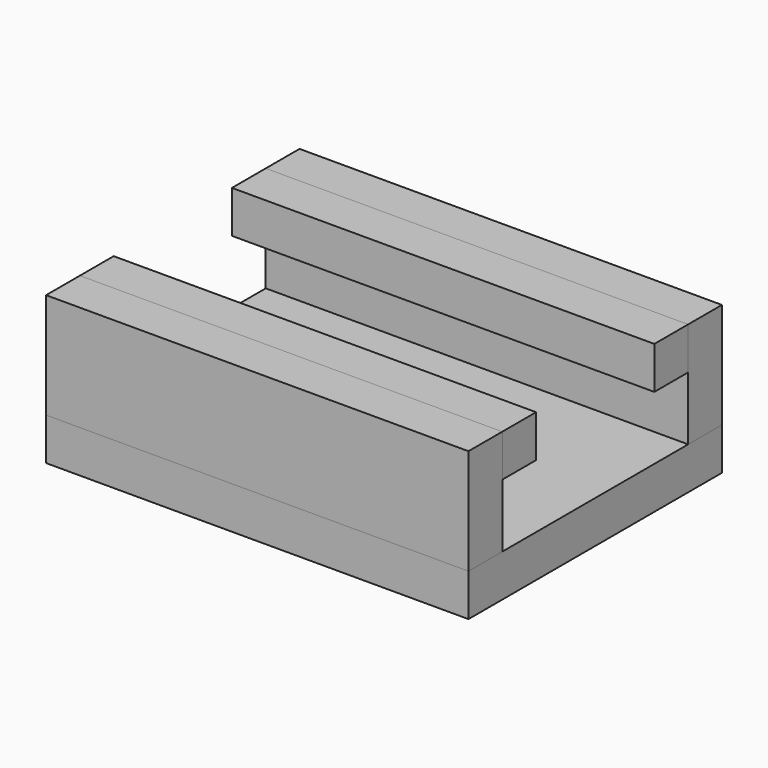
from build123d import *

# Parameters (mm, degrees)
F0_W     = 20
F0_H     = 2
F1_DEPTH = 7
F0_H_2   = 7
F2_DEPTH = 2
F3_START = 5
F3_DEPTH = 2


with BuildPart() as f1:
    # F0 (on Top) → F1 (new body)
    with BuildSketch(Plane.XY):
        with Locations((-33.0076411562, -6.5)):
            Rectangle(F0_W, F0_H)
    extrude(amount=F1_DEPTH)


with BuildPart() as f1b:
    # F0 (on Top) → F1, piece 2 (new body)
    with BuildSketch(Plane.XY):
        with Locations((-33.0076411562, 6.5)):
            Rectangle(F0_W, F0_H)
    extrude(amount=F1_DEPTH)


with BuildPart() as f2:
    # F0 (on Top) → F2 (new body)
    with BuildSketch(Plane.XY):
        with Locations((-33.0076411562, 6.5)):
            Rectangle(F0_W, F0_H)
        with Locations((-33.0076411562, 4.5)):
            Rectangle(F0_W, F0_H)
        with Locations((-33.0076411562, 0)):
            Rectangle(F0_W, F0_H_2)
        with Locations((-33.0076411562, -4.5)):
            Rectangle(F0_W, F0_H)
        with Locations((-33.0076411562, -6.5)):
            Rectangle(F0_W, F0_H)
    extrude(amount=F2_DEPTH)


with BuildPart() as f3:
    # F0 (on Top) → F3 (new body)
    with BuildSketch(Plane.XY.offset(F3_START)):
        with Locations((-33.0076411562, 4.5)):
            Rectangle(F0_W, F0_H)
    extrude(amount=F3_DEPTH)


with BuildPart() as f3b:
    # F0 (on Top) → F3, piece 2 (new body)
    with BuildSketch(Plane.XY.offset(F3_START)):
        with Locations((-33.0076411562, -4.5)):
            Rectangle(F0_W, F0_H)
    extrude(amount=F3_DEPTH)


solid = Compound([f1.part, f1b.part, f2.part, f3.part, f3b.part])
